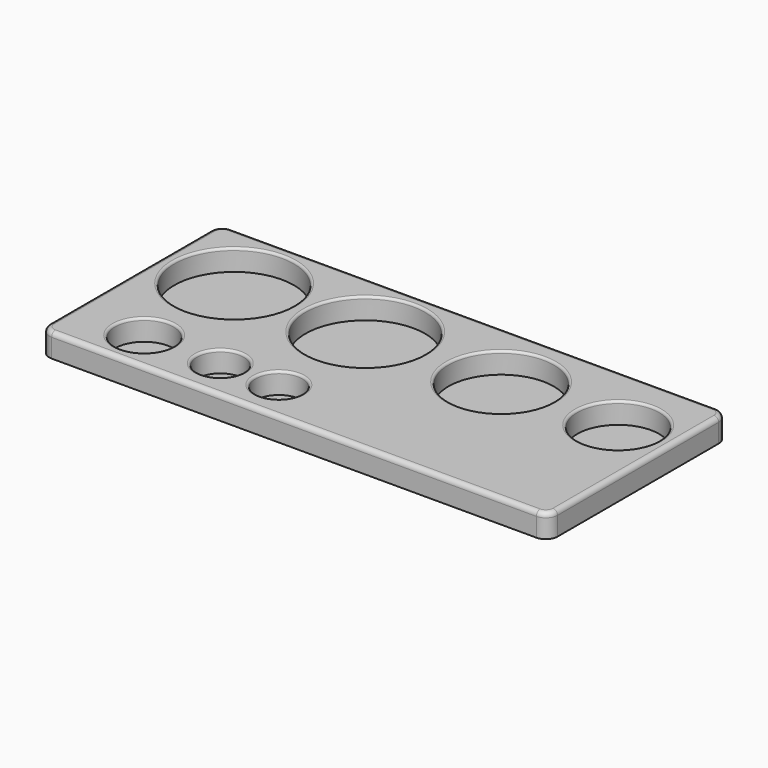
from build123d import *

# Parameters (mm, degrees)
F0_W         = 217
F0_H         = 96
F0_R         = 12.5
F0_R_2       = 10
F0_R_3       = 25.5
F0_R_4       = 22.5
F0_R_5       = 17.5
F1_DEPTH     = 10
F2_DEPTH     = 1
F3_R         = 1
F4_R         = 2
F5_T1_DEPTH  = 22.5
F5_T4_ANGLE  = 90
F5_T6_ANGLE  = 90
F5_T8_ANGLE  = 90
F5_T10_ANGLE = 90


# Not quite as in the source:
# - a fillet or chamfer that OpenCascade refuses, or shapes differently, is made with other operations: its cross-section is extruded or revolved along the edge and cut away or added


with BuildPart() as f1:
    # F0 (on Top) → F1 (new body)
    with BuildSketch(Plane.XY):
        Rectangle(F0_W, F0_H)
        with Locations((-78, -30.5)):
            Circle(F0_R, mode=Mode.SUBTRACT)
        with Locations((-45.5, -30.5)):
            Circle(F0_R_2, mode=Mode.SUBTRACT)
        with Locations((-20.5, -30.5)):
            Circle(F0_R_2, mode=Mode.SUBTRACT)
        with Locations((-78, 17.5)):
            Circle(F0_R_3, mode=Mode.SUBTRACT)
        with Locations((-22, 17.5)):
            Circle(F0_R_3, mode=Mode.SUBTRACT)
        with Locations((36, 17.5)):
            Circle(F0_R_4, mode=Mode.SUBTRACT)
        with Locations((86, 17.5)):
            Circle(F0_R_5, mode=Mode.SUBTRACT)
    extrude(amount=F1_DEPTH)

    # F0 (on Top) → F2 (join)
    with BuildSketch(Plane.XY):
        with Locations((-78, 17.5)):
            Circle(F0_R_3)
        with Locations((-22, 17.5)):
            Circle(F0_R_3)
        with Locations((36, 17.5)):
            Circle(F0_R_4)
        with Locations((86, 17.5)):
            Circle(F0_R_5)
        with Locations((-78, -30.5)):
            Circle(F0_R)
        with Locations((-45.5, -30.5)):
            Circle(F0_R_2)
        with Locations((-20.5, -30.5)):
            Circle(F0_R_2)
    extrude(amount=F2_DEPTH)

    # F3
    f3_edges = [f1.edges().sort_by_distance(p)[0] for p in [
        (-103.5, 17.5, 10),
        (-47.5, 17.5, 10),
        (13.5, 17.5, 10),
        (68.5, 17.5, 10),
        (-90.5, -30.5, 10),
        (-55.5, -30.5, 10),
        (-30.5, -30.5, 10),
    ]]
    fillet(f3_edges, radius=F3_R)

    # F4
    f4_edges = [f1.edges().sort_by_distance(p)[0] for p in [
        (-108.5, 0, 10),
        (0, 48, 10),
        (108.5, 0, 10),
        (0, -48, 10),
    ]]
    fillet(f4_edges, radius=F4_R)

    # F5: fillet of radius 5 on 8 edges, made by hand

    # F5_s2 → F5_t1 (cut)
    with BuildSketch(Plane.XY.offset(-12.5)):
        with BuildLine():
            ThreePointArc((-108.5, -43), (-107.0355339059, -46.5355339059), (-103.5, -48))
            Line((-103.5, -48), (-108.5, -48))
            Line((-108.5, -48), (-108.5, -43))
        make_face()
        with BuildLine():
            ThreePointArc((-108.5, 43), (-107.0355339059, 46.5355339059), (-103.5, 48))
            Line((-103.5, 48), (-108.5, 48))
            Line((-108.5, 48), (-108.5, 43))
        make_face()
        with BuildLine():
            ThreePointArc((103.5, 48), (107.0355339059, 46.5355339059), (108.5, 43))
            Line((108.5, 43), (108.5, 48))
            Line((108.5, 48), (103.5, 48))
        make_face()
        with BuildLine():
            ThreePointArc((103.5, -48), (107.0355339059, -46.5355339059), (108.5, -43))
            Line((108.5, -43), (108.5, -48))
            Line((108.5, -48), (103.5, -48))
        make_face()
    extrude(amount=F5_T1_DEPTH, mode=Mode.SUBTRACT)

    # F5_s3 → F5_t4 (revolve, cut)
    with BuildSketch(Plane.XZ.offset(43)):
        with BuildLine():
            ThreePointArc((-106.5, 10), (-107.9142135624, 9.4142135624), (-108.5, 8))
            Line((-108.5, 8), (-108.5, 10))
            Line((-108.5, 10), (-106.5, 10))
        make_face()
    revolve(axis=Axis((-103.5, -43, 10), (0, 0, 1)), revolution_arc=F5_T4_ANGLE, mode=Mode.SUBTRACT)

    # F5_s5 → F5_t6 (revolve, cut)
    with BuildSketch(Plane.YZ.offset(-103.5)):
        with BuildLine():
            ThreePointArc((46, 10), (47.4142135624, 9.4142135624), (48, 8))
            Line((48, 8), (48, 10))
            Line((48, 10), (46, 10))
        make_face()
    revolve(axis=Axis((-103.5, 43, 10), (0, 0, 1)), revolution_arc=F5_T6_ANGLE, mode=Mode.SUBTRACT)

    # F5_s7 → F5_t8 (revolve, cut)
    with BuildSketch(Plane.XZ.offset(-43)):
        with BuildLine():
            ThreePointArc((106.5, 10), (107.9142135624, 9.4142135624), (108.5, 8))
            Line((108.5, 8), (108.5, 10))
            Line((108.5, 10), (106.5, 10))
        make_face()
    revolve(axis=Axis((103.5, 43, 10), (0, 0, 1)), revolution_arc=F5_T8_ANGLE, mode=Mode.SUBTRACT)

    # F5_s9 → F5_t10 (revolve, cut)
    with BuildSketch(Plane.YZ.offset(103.5)):
        with BuildLine():
            ThreePointArc((-46, 10), (-47.4142135624, 9.4142135624), (-48, 8))
            Line((-48, 8), (-48, 10))
            Line((-48, 10), (-46, 10))
        make_face()
    revolve(axis=Axis((103.5, -43, 10), (0, 0, 1)), revolution_arc=F5_T10_ANGLE, mode=Mode.SUBTRACT)


solid = f1.part
